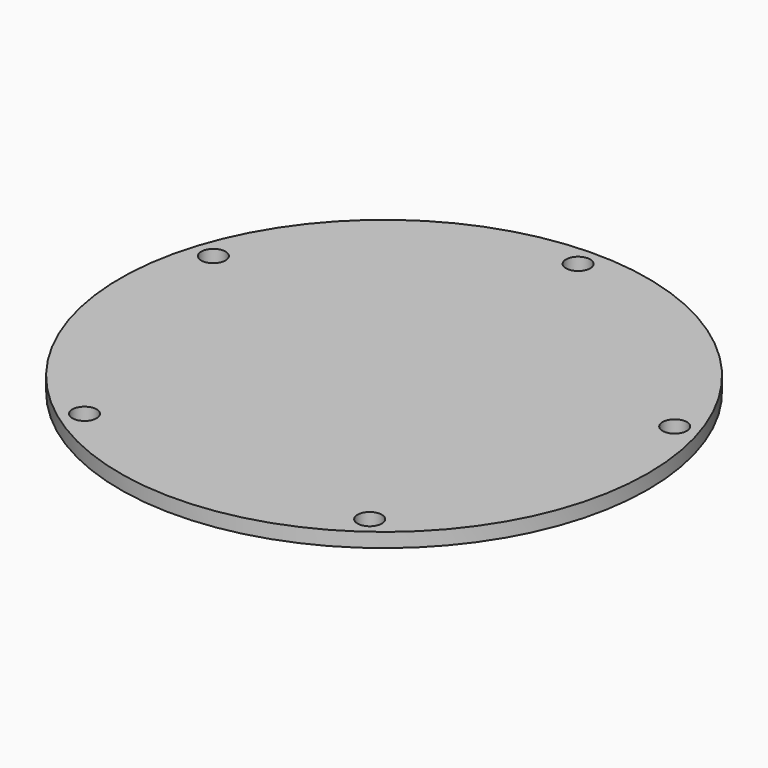
from build123d import *

# Parameters (mm, degrees)
F0_R     = 92.5
F0_R_2   = 4.25
F1_DEPTH = 5


# Not quite as in the source:
# - a feature names something its author has since deleted; it is built from what else it names


with BuildPart() as f1:
    # F0 (on Top) → F1 (new body)
    with BuildSketch(Plane.XY):
        Circle(F0_R)
        with Locations((-49.9617464449, -68.7664445219)):
            Circle(F0_R_2, mode=Mode.SUBTRACT)
        with Locations((49.9617464449, -68.7664445219)):
            Circle(F0_R_2, mode=Mode.SUBTRACT)
        with Locations((-80.8398038851, 26.2664445219)):
            Circle(F0_R_2, mode=Mode.SUBTRACT)
        with Locations((80.8398038851, 26.2664445219)):
            Circle(F0_R_2, mode=Mode.SUBTRACT)
        with Locations((0, 85)):
            Circle(F0_R_2, mode=Mode.SUBTRACT)
    extrude(amount=F1_DEPTH)


solid = f1.part
